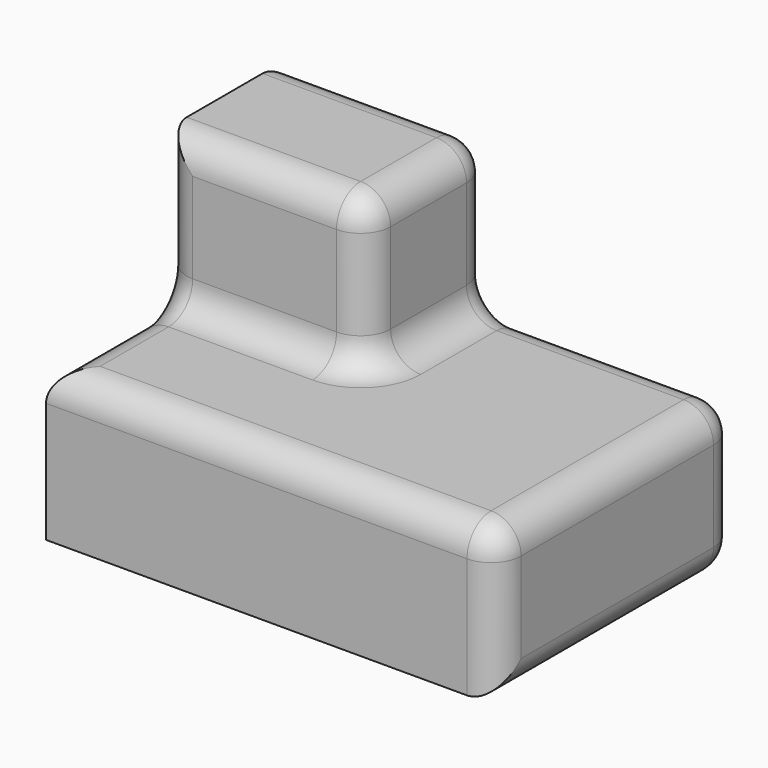
from build123d import *

# Parameters (mm, degrees)
F0_W     = 76.2
F0_H     = 50.8
F1_DEPTH = 25.4
F2_W     = 34.4617506489
F2_H     = 26.1815364093
F3_DEPTH = 25.4
F4_R     = 5.08


with BuildPart() as f1:
    # F0 (on Top) → F1 (new body)
    with BuildSketch(Plane.XY):
        with Locations((14.1653842241, 0.7815364093)):
            Rectangle(F0_W, F0_H)
    extrude(amount=F1_DEPTH)

    # F2 (on face) → F3 (join)
    with BuildSketch(Plane.XY.offset(25.4)):
        with Locations((-6.7037404515, 13.0907682046)):
            Rectangle(F2_W, F2_H)
    extrude(amount=F3_DEPTH)

    # F4
    f4_edges = [f1.edges().sort_by_distance(p)[0] for p in [
        (-6.70374, 0, 25.4),
        (10.527135, 13.090768, 25.4),
        (14.165384, -24.618464, 25.4),
        (52.265384, 0.781536, 25.4),
        (52.265384, -24.618464, 12.7),
        (52.265384, 26.181536, 12.7),
        (52.265384, 0.781536, 0),
        (14.165384, 26.181536, 0),
        (31.39626, 26.181536, 25.4),
        (-6.70374, 26.181536, 50.8),
        (-23.934616, 26.181536, 25.4),
        (10.527135, 13.090768, 50.8),
        (-6.70374, 0, 50.8),
        (-23.934616, 0, 38.1),
        (10.527135, 0, 38.1),
        (10.527135, 26.181536, 38.1),
        (-23.934616, -12.309232, 25.4),
    ]]
    fillet(f4_edges, radius=F4_R)


solid = f1.part
